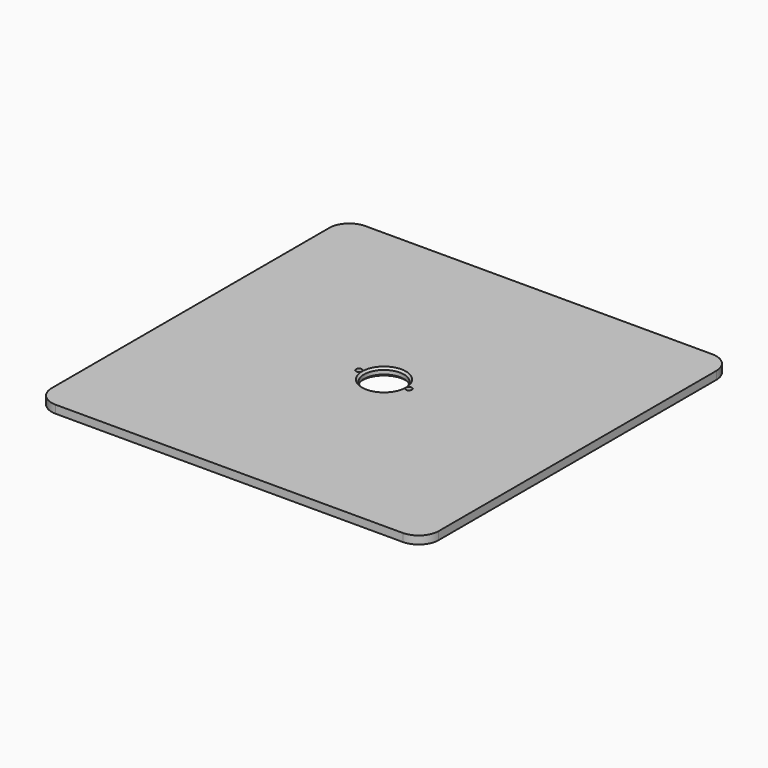
from build123d import *

# Parameters (mm, degrees)
F0_W     = 194
F0_H     = 194
F0_R     = 1.5
F0_R_2   = 10
F1_DEPTH = 4
F2_SIZE  = 0.99999
F3_R     = 10


# Not quite as in the source:
# - a fillet or chamfer is up to 0.001 mm smaller than in the source, because OpenCascade refuses the exact size


with BuildPart() as f1:
    # F0 (on Top) → F1 (new body)
    with BuildSketch(Plane.XY):
        Rectangle(F0_W, F0_H)
        with Locations((-12.5, 0)):
            Circle(F0_R, mode=Mode.SUBTRACT)
        Circle(F0_R_2, mode=Mode.SUBTRACT)
        with Locations((12.5, 0)):
            Circle(F0_R, mode=Mode.SUBTRACT)
    extrude(amount=F1_DEPTH)

    # F2 (size 1 in the source; OpenCascade refuses exactly that, so slightly less here)
    f2_edges = [f1.edges().sort_by_distance(p)[0] for p in [
        (-10, 0, 4),
        (-10, 0, 0),
    ]]
    chamfer(f2_edges, length=F2_SIZE)

    # F3
    f3_edges = [f1.edges().sort_by_distance(p)[0] for p in [
        (-97, 97, 2),
        (-97, -97, 2),
        (97, -97, 2),
        (97, 97, 2),
    ]]
    fillet(f3_edges, radius=F3_R)


solid = f1.part
